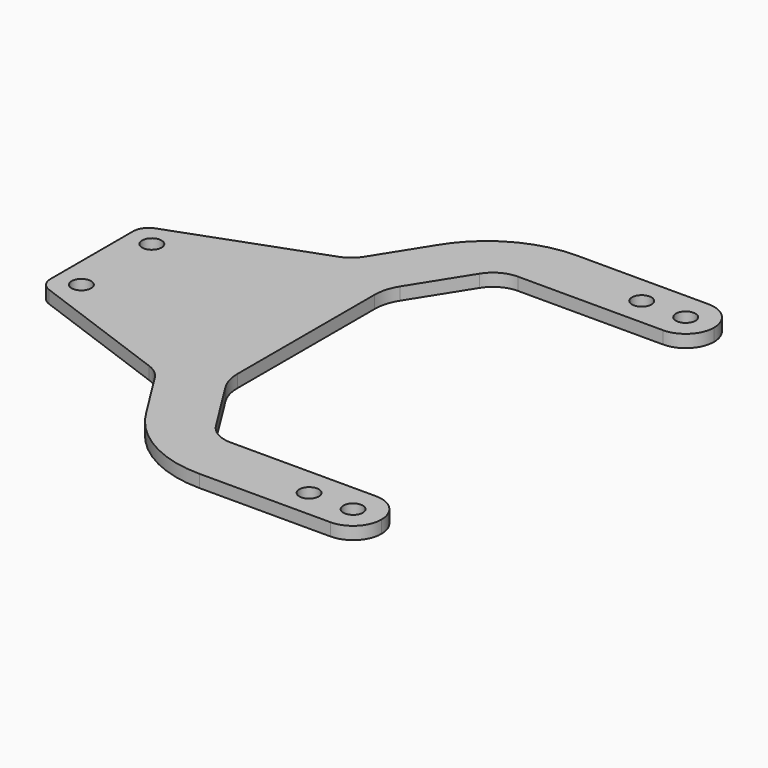
from build123d import *

# Parameters (mm, degrees)
F0_R     = 1.55
F1_DEPTH = 2


# Not quite as in the source:
# - a feature names something its author has since deleted; it is built from what else it names


with BuildPart() as f1:
    # F0 (on Top) → F1 (new body)
    with BuildSketch(Plane.XY):
        with BuildLine():
            Line((25.4436091884, 28.55), (48.5000015985, 28.55))
            ThreePointArc((48.5000015985, 28.55), (51.6819821139, 29.8680194847), (53.0000015985, 33.05))
            ThreePointArc((53.0000015985, 33.05), (51.6819821139, 36.2319805153), (48.5000015985, 37.55))
            Line((48.5000015985, 37.55), (27.6442359668, 37.55))
            ThreePointArc((27.6442359668, 37.55), (18.7122132684, 35.1775068554), (12.1347641944, 28.6854411684))
            Line((12.1347641944, 28.6854411684), (7.2011388972, 20.8408842798))
            ThreePointArc((7.2011388972, 20.8408842798), (6.1134719977, 19.6156574256), (4.6881494145, 18.8077863577))
            Line((4.6881494145, 18.8077863577), (-17.8597609739, 10.5497599571))
            ThreePointArc((-17.8597609739, 10.5497599571), (-19.0493172564, 9.6341347233), (-19.5, 8.2022482814))
            Line((-19.5, 8.2022482814), (-19.5, -8.2022482814))
            ThreePointArc((-19.5, -8.2022482814), (-19.0493172564, -9.6341347233), (-17.8597609739, -10.5497599571))
            Line((-17.8597609739, -10.5497599571), (4.6881494145, -18.8077863577))
            ThreePointArc((4.6881494145, -18.8077863577), (6.1134719977, -19.6156574256), (7.2011388972, -20.8408842798))
            Line((7.2011388972, -20.8408842798), (12.1347641944, -28.6854411684))
            ThreePointArc((12.1347641944, -28.6854411684), (18.7122132684, -35.1775068554), (27.6442359668, -37.55))
            Line((27.6442359668, -37.55), (48.5000015985, -37.55))
            ThreePointArc((48.5000015985, -37.55), (51.6819821139, -36.2319805153), (53.0000015985, -33.05))
            ThreePointArc((53.0000015985, -33.05), (51.6819821139, -29.8680194847), (48.5000015985, -28.55))
            Line((48.5000015985, -28.55), (25.4436091884, -28.55))
            ThreePointArc((25.4436091884, -28.55), (23.0259271525, -27.9266212509), (21.211097758, -26.2119254294))
            Line((21.211097758, -26.2119254294), (15.6422879472, -17.3574132338))
            ThreePointArc((15.6422879472, -17.3574132338), (14.8417868513, -15.5699685166), (14.5678039498, -13.6307176327))
            Line((14.5678039498, -13.6307176327), (14.5678039498, 13.6307176327))
            ThreePointArc((14.5678039498, 13.6307176327), (14.8417868513, 15.5699685166), (15.6422879472, 17.3574132338))
            Line((15.6422879472, 17.3574132338), (21.211097758, 26.2119254294))
            ThreePointArc((21.211097758, 26.2119254294), (23.0259271525, 27.9266212509), (25.4436091884, 28.55))
        make_face()
        with Locations((-15.55, -7)):
            Circle(F0_R, mode=Mode.SUBTRACT)
        with Locations((41.5000015985, -33.05)):
            Circle(F0_R, mode=Mode.SUBTRACT)
        with Locations((48.5000015985, -33.05)):
            Circle(F0_R, mode=Mode.SUBTRACT)
        with Locations((-15.55, 7)):
            Circle(F0_R, mode=Mode.SUBTRACT)
        with Locations((41.5000015985, 33.05)):
            Circle(F0_R, mode=Mode.SUBTRACT)
        with Locations((48.5000015985, 33.05)):
            Circle(F0_R, mode=Mode.SUBTRACT)
    extrude(amount=F1_DEPTH)


solid = f1.part
